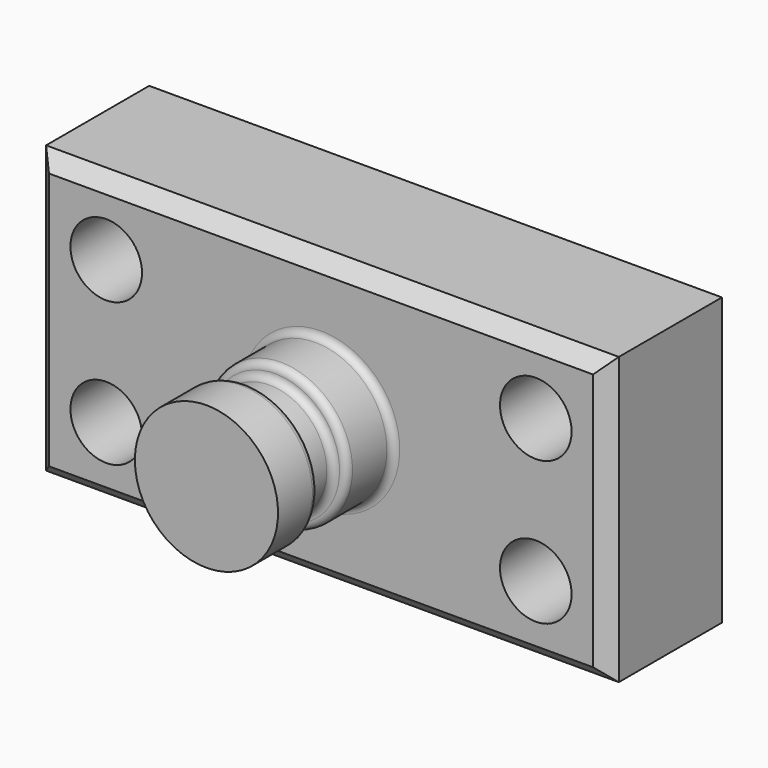
from build123d import *

# Parameters (mm, degrees)
F0_W     = 101.6
F0_H     = 50.8
F1_DEPTH = 25.4
F2_R     = 6.35
F3_DEPTH = 25.401
F4_W     = 12.7
F4_H     = 25.4
F6_W     = 6.9762246056
F6_H     = 6.35
F8_R     = 1.26999
F9_SIZE  = 2.54


# Not quite as in the source:
# - a fillet or chamfer is up to 0.001 mm smaller than in the source, because OpenCascade refuses the exact size


with BuildPart() as f1:
    # F0 (on Front) → F1 (new body)
    with BuildSketch(Plane.XZ):
        Rectangle(F0_W, F0_H)
    extrude(amount=F1_DEPTH)

    # F2 (on face) → F3 (cut, through all)
    with BuildSketch(Plane.XZ.offset(25.4)):
        with Locations((-38.1, 12.7)):
            Circle(F2_R)
        with Locations((-38.1, -12.7)):
            Circle(F2_R)
        with Locations((38.1, -12.7)):
            Circle(F2_R)
        with Locations((38.1, 12.7)):
            Circle(F2_R)
    extrude(amount=-F3_DEPTH, mode=Mode.SUBTRACT)

    # F4 (on Top) → F5 (revolve)
    with BuildSketch(Plane.XY):
        with Locations((-6.35, -38.1)):
            Rectangle(F4_W, F4_H)
    revolve(axis=Axis((0, -38.1, 0), (0, -1, 0)))

    # F6 (on Top) → F7 (revolve, cut)
    with BuildSketch(Plane.XY):
        with Locations((-13.6481123028, -38.735)):
            Rectangle(F6_W, F6_H)
    revolve(axis=Axis((0, -32.9395644367, 0), (0, -1, 0)), mode=Mode.SUBTRACT)

    # F8 (radius 1.27 in the source; OpenCascade refuses exactly that, so slightly less here)
    f8_edges = [f1.edges().sort_by_distance(p)[0] for p in [
        (12.7, -25.4, 0),
        (10.16, -41.91, 0),
        (10.16, -35.56, 0),
        (12.7, -41.91, 0),
        (12.7, -35.56, 0),
    ]]
    fillet(f8_edges, radius=F8_R)

    # F9
    f9_edges = [f1.edges().sort_by_distance(p)[0] for p in [
        (0, -25.4, -25.4),
        (-50.8, -25.4, 0),
        (0, -25.4, 25.4),
        (50.8, -25.4, 0),
    ]]
    chamfer(f9_edges, length=F9_SIZE)


solid = f1.part
